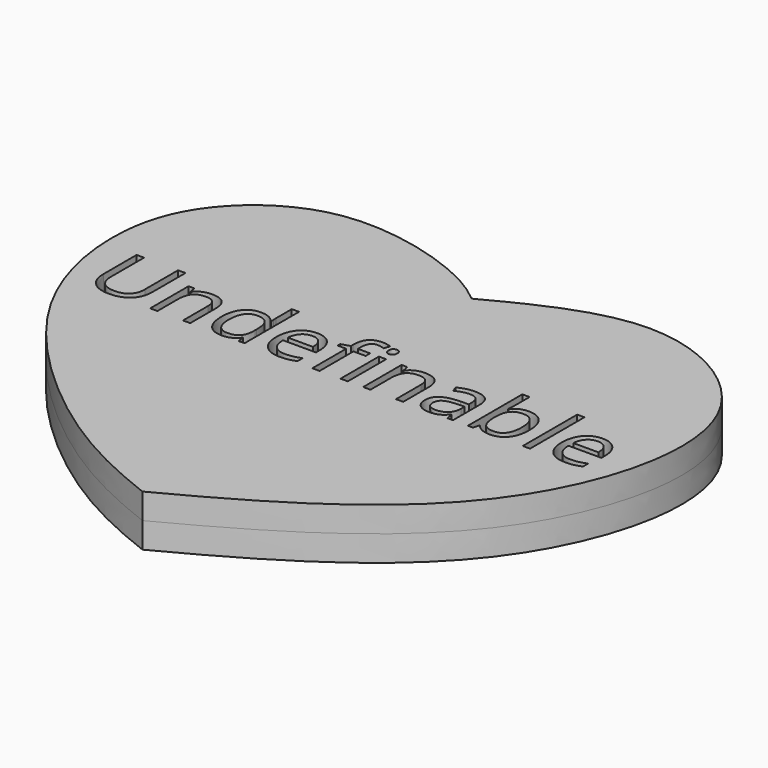
from build123d import *

# Parameters (mm, degrees)
F1_DEPTH     = 4
F2_SCALE     = 0.5
F3_TEXT_SIZE = 6.9970207997
F4_DEPTH     = 3


# Not quite as in the source:
# - Text() gives the source's letters only with a copy of the font that has no kerning and outlines rounded to 1/6400 em; it was checked with that copy


with BuildPart() as f1:
    # F0 (on Top) → F1 (new body, symmetric)
    with BuildSketch(Plane.XY):
        with BuildLine():
            add(Edge.make_bspline(
                [(49.6034175158, 70.3383758664), (57.4255755938, 74.4701894092), (72.777071302, 82.1686280864), (98.5809075936, 66.4625184016), (89.6533310415, 28.6744955736), (66.9245487128, 14.178657317), (50.0742010772, 5.4191295058)],
                knots=[0, 0, 0, 0, 0.2245214689, 0.4410611027, 0.6922062561, 1, 1, 1, 1], degree=3))
            add(Edge.make_bspline(
                [(49.6034175158, 70.3383758664), (47.4339338141, 72.2192165566), (41.0433747036, 76.0012562734), (22.277013048, 80.0594704424), (7.7702176976, 69.6318815381), (3.9007087353, 55.4213262189), (8.818104806, 34.6134665552), (31.3463892668, 13.6516026811), (43.7721535607, 7.8800658319), (50.0742010772, 5.4191295058)],
                knots=[0, 0, 0, 0, 0.106242303, 0.2507252939, 0.3862136345, 0.5102499506, 0.6625335349, 0.8471651701, 1, 1, 1, 1], degree=3))
        make_face()
    extrude(amount=F1_DEPTH, both=True)


with BuildPart() as f1_1:
    # F2: moved
    add(f1.part.scale(F2_SCALE))

    # F3 (on Top) → F4 (cut)
    with BuildSketch(Plane.XY):
        with Locations((4.590751593, 21.9124035204)):
            Text('Undefinable', F3_TEXT_SIZE, font='Open Sans', text_align=(TextAlign.LEFT, TextAlign.BOTTOM))
    extrude(amount=F4_DEPTH, mode=Mode.SUBTRACT)


solid = f1_1.part
